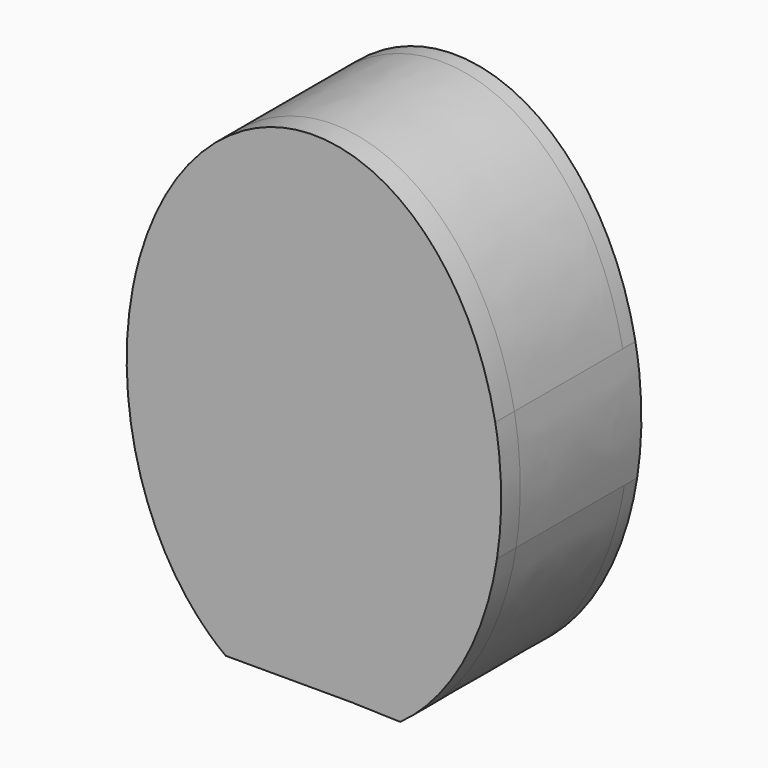
from build123d import *

# Parameters (mm, degrees)
F1_DEPTH = 2
F2_START = 2
F2_DEPTH = 17
F3_START = 19
F3_DEPTH = 3
F4_DEPTH = 22
F5_DEPTH = 1.9


# Not quite as in the source:
# - a feature names something its author has since deleted; it is built from what else it names


with BuildPart() as f1:
    # F0 (on Front) → F1 (new body)
    with BuildSketch(Plane.XZ):
        with BuildLine():
            ThreePointArc((22.615939659, -28.955879261), (25.4430057238, -23.4443332064), (29.5330586852, -18.7923541416))
            ThreePointArc((29.5330586852, -18.7923541416), (31.5285740741, -1.0914136246), (14.5694942222, 4.3578971054))
            ThreePointArc((14.5694942222, 4.3578971054), (10.2295706847, 0.7277849341), (6.5230501824, -3.5470666953))
            ThreePointArc((6.5230501824, -3.5470666953), (5.0741774638, -5.5394834496), (4.0740678087, -7.7908691019))
            ThreePointArc((4.0740678087, -7.7908691019), (2.9738142449, -8.0303676706), (2.3612100631, -7.0855747908))
            ThreePointArc((2.3612100631, -7.0855747908), (3.4264007601, -4.0400208243), (5.1113933333, -1.2885066571))
            ThreePointArc((5.1113933333, -1.2885066571), (8.6689265704, 3.4029198706), (13.299004455, 7.0399384822))
            ThreePointArc((13.299004455, 7.0399384822), (32.0541613054, 3.3946614198), (36.1678472728, -15.2633540456))
            ThreePointArc((36.1678472728, -15.2633540456), (31.3626226074, -22.0360379057), (26.9920754255, -29.0970398237))
            ThreePointArc((26.9920754255, -29.0970398237), (25.2131477889, -37.6146832372), (25.5804176451, -46.3083559771))
            Line((25.5804176451, -46.3083559771), (31.5964009875, -46.4919595582))
            add(Edge.make_bspline(
                [(31.5964009875, -46.4919595582), (41.4151881919, -39.4487656176), (43.7491179336, -24.5017576963)],
                knots=[0.4786752717, 0.4786752717, 0.4786752717, 1.3582145289, 1.3582145289, 1.3582145289], degree=2, weights=[1, 0.9048497635, 1]))
            Line((43.7491179336, -24.5017576963), (41.5137453779, -24.5017576963))
            Line((41.5137453779, -24.5017576963), (40.8978872001, -24.5017576963))
            Line((40.8978872001, -24.5017576963), (40.8978872001, -9.5017576963))
            Line((40.8978872001, -9.5017576963), (41.4988510311, -9.5017576963))
            Line((41.4988510311, -9.5017576963), (43.5284191526, -9.5017576963))
            add(Edge.make_bspline(
                [(43.5284191526, -9.5017576963), (38.9680565578, 14.8552314192), (20.7669530064, 14.8552314192), (2.5658494549, 14.8552314192), (-1.9945131398, -9.5017576963)],
                knots=[1.82404898, 1.82404898, 1.82404898, 3.1415926536, 3.1415926536, 4.4591363272, 4.4591363272, 4.4591363272], degree=2, weights=[1, 0.7907446431, 1, 0.7907446431, 1]))
            Line((-1.9945131398, -9.5017576963), (0, -9.5017576963))
            Line((0, -9.5017576963), (0.8074482903, -9.5017576963))
            Line((0.8074482903, -9.5017576963), (0.8074482903, -24.5017576963))
            Line((0.8074482903, -24.5017576963), (0, -24.5017576963))
            Line((0, -24.5017576963), (-2.2152119208, -24.5017576963))
            add(Edge.make_bspline(
                [(-2.2152119208, -24.5017576963), (0.0820950249, -39.2142250435), (9.6852980207, -46.3083559771)],
                knots=[4.9249707783, 4.9249707783, 4.9249707783, 5.7923862825, 5.7923862825, 5.7923862825], degree=2, weights=[1, 0.9074138517, 1]))
            Line((9.6852980207, -46.3083559771), (21.2042818786, -46.3083559771))
            ThreePointArc((21.2042818786, -46.3083559771), (21.3694737395, -37.5881357437), (22.615939659, -28.955879261))
        make_face()
        with BuildLine():
            ThreePointArc((14.5694942222, 4.3578971054), (31.5285740741, -1.0914136246), (29.5330586852, -18.7923541416))
            ThreePointArc((29.5330586852, -18.7923541416), (25.4430057238, -23.4443332064), (22.615939659, -28.955879261))
            ThreePointArc((22.615939659, -28.955879261), (21.3694737395, -37.5881357437), (21.2042818786, -46.3083559771))
            Line((21.2042818786, -46.3083559771), (25.5804176451, -46.3083559771))
            ThreePointArc((25.5804176451, -46.3083559771), (25.2131477889, -37.6146832372), (26.9920754255, -29.0970398237))
            ThreePointArc((26.9920754255, -29.0970398237), (31.3626226074, -22.0360379057), (36.1678472728, -15.2633540456))
            ThreePointArc((36.1678472728, -15.2633540456), (32.0541613054, 3.3946614198), (13.299004455, 7.0399384822))
            ThreePointArc((13.299004455, 7.0399384822), (8.6689265704, 3.4029198706), (5.1113933333, -1.2885066571))
            ThreePointArc((5.1113933333, -1.2885066571), (3.4264007601, -4.0400208243), (2.3612100631, -7.0855747908))
            ThreePointArc((2.3612100631, -7.0855747908), (2.9738142449, -8.0303676706), (4.0740678087, -7.7908691019))
            ThreePointArc((4.0740678087, -7.7908691019), (5.0741774638, -5.5394834496), (6.5230501824, -3.5470666953))
            ThreePointArc((6.5230501824, -3.5470666953), (10.2295706847, 0.7277849341), (14.5694942222, 4.3578971054))
        make_face()
    extrude(amount=F1_DEPTH)

    # F0 (on Front) → F2 (join)
    with BuildSketch(Plane.XZ.offset(F2_START)):
        with BuildLine():
            ThreePointArc((22.615939659, -28.955879261), (25.4430057238, -23.4443332064), (29.5330586852, -18.7923541416))
            ThreePointArc((29.5330586852, -18.7923541416), (31.5285740741, -1.0914136246), (14.5694942222, 4.3578971054))
            ThreePointArc((14.5694942222, 4.3578971054), (10.2295706847, 0.7277849341), (6.5230501824, -3.5470666953))
            ThreePointArc((6.5230501824, -3.5470666953), (5.0741774638, -5.5394834496), (4.0740678087, -7.7908691019))
            ThreePointArc((4.0740678087, -7.7908691019), (2.9738142449, -8.0303676706), (2.3612100631, -7.0855747908))
            ThreePointArc((2.3612100631, -7.0855747908), (3.4264007601, -4.0400208243), (5.1113933333, -1.2885066571))
            ThreePointArc((5.1113933333, -1.2885066571), (8.6689265704, 3.4029198706), (13.299004455, 7.0399384822))
            ThreePointArc((13.299004455, 7.0399384822), (32.0541613054, 3.3946614198), (36.1678472728, -15.2633540456))
            ThreePointArc((36.1678472728, -15.2633540456), (31.3626226074, -22.0360379057), (26.9920754255, -29.0970398237))
            ThreePointArc((26.9920754255, -29.0970398237), (25.2131477889, -37.6146832372), (25.5804176451, -46.3083559771))
            Line((25.5804176451, -46.3083559771), (31.5964009875, -46.4919595582))
            add(Edge.make_bspline(
                [(31.5964009875, -46.4919595582), (41.4151881919, -39.4487656176), (43.7491179336, -24.5017576963)],
                knots=[0.4786752717, 0.4786752717, 0.4786752717, 1.3582145289, 1.3582145289, 1.3582145289], degree=2, weights=[1, 0.9048497635, 1]))
            Line((43.7491179336, -24.5017576963), (41.5137453779, -24.5017576963))
            Line((41.5137453779, -24.5017576963), (40.8978872001, -24.5017576963))
            Line((40.8978872001, -24.5017576963), (40.8978872001, -9.5017576963))
            Line((40.8978872001, -9.5017576963), (41.4988510311, -9.5017576963))
            Line((41.4988510311, -9.5017576963), (43.5284191526, -9.5017576963))
            add(Edge.make_bspline(
                [(43.5284191526, -9.5017576963), (38.9680565578, 14.8552314192), (20.7669530064, 14.8552314192), (2.5658494549, 14.8552314192), (-1.9945131398, -9.5017576963)],
                knots=[1.82404898, 1.82404898, 1.82404898, 3.1415926536, 3.1415926536, 4.4591363272, 4.4591363272, 4.4591363272], degree=2, weights=[1, 0.7907446431, 1, 0.7907446431, 1]))
            Line((-1.9945131398, -9.5017576963), (0, -9.5017576963))
            Line((0, -9.5017576963), (0.8074482903, -9.5017576963))
            Line((0.8074482903, -9.5017576963), (0.8074482903, -24.5017576963))
            Line((0.8074482903, -24.5017576963), (0, -24.5017576963))
            Line((0, -24.5017576963), (-2.2152119208, -24.5017576963))
            add(Edge.make_bspline(
                [(-2.2152119208, -24.5017576963), (0.0820950249, -39.2142250435), (9.6852980207, -46.3083559771)],
                knots=[4.9249707783, 4.9249707783, 4.9249707783, 5.7923862825, 5.7923862825, 5.7923862825], degree=2, weights=[1, 0.9074138517, 1]))
            Line((9.6852980207, -46.3083559771), (21.2042818786, -46.3083559771))
            ThreePointArc((21.2042818786, -46.3083559771), (21.3694737395, -37.5881357437), (22.615939659, -28.955879261))
        make_face()
    extrude(amount=F2_DEPTH)


with BuildPart() as f3:
    # F0 (on Front) → F3 (new body)
    with BuildSketch(Plane.XZ.offset(F3_START)):
        with BuildLine():
            ThreePointArc((22.615939659, -28.955879261), (25.4430057238, -23.4443332064), (29.5330586852, -18.7923541416))
            ThreePointArc((29.5330586852, -18.7923541416), (31.5285740741, -1.0914136246), (14.5694942222, 4.3578971054))
            ThreePointArc((14.5694942222, 4.3578971054), (10.2295706847, 0.7277849341), (6.5230501824, -3.5470666953))
            ThreePointArc((6.5230501824, -3.5470666953), (5.0741774638, -5.5394834496), (4.0740678087, -7.7908691019))
            ThreePointArc((4.0740678087, -7.7908691019), (2.9738142449, -8.0303676706), (2.3612100631, -7.0855747908))
            ThreePointArc((2.3612100631, -7.0855747908), (3.4264007601, -4.0400208243), (5.1113933333, -1.2885066571))
            ThreePointArc((5.1113933333, -1.2885066571), (8.6689265704, 3.4029198706), (13.299004455, 7.0399384822))
            ThreePointArc((13.299004455, 7.0399384822), (32.0541613054, 3.3946614198), (36.1678472728, -15.2633540456))
            ThreePointArc((36.1678472728, -15.2633540456), (31.3626226074, -22.0360379057), (26.9920754255, -29.0970398237))
            ThreePointArc((26.9920754255, -29.0970398237), (25.2131477889, -37.6146832372), (25.5804176451, -46.3083559771))
            Line((25.5804176451, -46.3083559771), (31.5964009875, -46.4919595582))
            add(Edge.make_bspline(
                [(31.5964009875, -46.4919595582), (41.4151881919, -39.4487656176), (43.7491179336, -24.5017576963)],
                knots=[0.4786752717, 0.4786752717, 0.4786752717, 1.3582145289, 1.3582145289, 1.3582145289], degree=2, weights=[1, 0.9048497635, 1]))
            Line((43.7491179336, -24.5017576963), (41.5137453779, -24.5017576963))
            Line((41.5137453779, -24.5017576963), (40.8978872001, -24.5017576963))
            Line((40.8978872001, -24.5017576963), (40.8978872001, -9.5017576963))
            Line((40.8978872001, -9.5017576963), (41.4988510311, -9.5017576963))
            Line((41.4988510311, -9.5017576963), (43.5284191526, -9.5017576963))
            add(Edge.make_bspline(
                [(43.5284191526, -9.5017576963), (38.9680565578, 14.8552314192), (20.7669530064, 14.8552314192), (2.5658494549, 14.8552314192), (-1.9945131398, -9.5017576963)],
                knots=[1.82404898, 1.82404898, 1.82404898, 3.1415926536, 3.1415926536, 4.4591363272, 4.4591363272, 4.4591363272], degree=2, weights=[1, 0.7907446431, 1, 0.7907446431, 1]))
            Line((-1.9945131398, -9.5017576963), (0, -9.5017576963))
            Line((0, -9.5017576963), (0.8074482903, -9.5017576963))
            Line((0.8074482903, -9.5017576963), (0.8074482903, -24.5017576963))
            Line((0.8074482903, -24.5017576963), (0, -24.5017576963))
            Line((0, -24.5017576963), (-2.2152119208, -24.5017576963))
            add(Edge.make_bspline(
                [(-2.2152119208, -24.5017576963), (0.0820950249, -39.2142250435), (9.6852980207, -46.3083559771)],
                knots=[4.9249707783, 4.9249707783, 4.9249707783, 5.7923862825, 5.7923862825, 5.7923862825], degree=2, weights=[1, 0.9074138517, 1]))
            Line((9.6852980207, -46.3083559771), (21.2042818786, -46.3083559771))
            ThreePointArc((21.2042818786, -46.3083559771), (21.3694737395, -37.5881357437), (22.615939659, -28.955879261))
        make_face()
        with BuildLine():
            ThreePointArc((14.5694942222, 4.3578971054), (31.5285740741, -1.0914136246), (29.5330586852, -18.7923541416))
            ThreePointArc((29.5330586852, -18.7923541416), (25.4430057238, -23.4443332064), (22.615939659, -28.955879261))
            ThreePointArc((22.615939659, -28.955879261), (21.3694737395, -37.5881357437), (21.2042818786, -46.3083559771))
            Line((21.2042818786, -46.3083559771), (25.5804176451, -46.3083559771))
            ThreePointArc((25.5804176451, -46.3083559771), (25.2131477889, -37.6146832372), (26.9920754255, -29.0970398237))
            ThreePointArc((26.9920754255, -29.0970398237), (31.3626226074, -22.0360379057), (36.1678472728, -15.2633540456))
            ThreePointArc((36.1678472728, -15.2633540456), (32.0541613054, 3.3946614198), (13.299004455, 7.0399384822))
            ThreePointArc((13.299004455, 7.0399384822), (8.6689265704, 3.4029198706), (5.1113933333, -1.2885066571))
            ThreePointArc((5.1113933333, -1.2885066571), (3.4264007601, -4.0400208243), (2.3612100631, -7.0855747908))
            ThreePointArc((2.3612100631, -7.0855747908), (2.9738142449, -8.0303676706), (4.0740678087, -7.7908691019))
            ThreePointArc((4.0740678087, -7.7908691019), (5.0741774638, -5.5394834496), (6.5230501824, -3.5470666953))
            ThreePointArc((6.5230501824, -3.5470666953), (10.2295706847, 0.7277849341), (14.5694942222, 4.3578971054))
        make_face()
        with BuildLine():
            Line((40.8978872001, -24.5017576963), (41.5137453779, -24.5017576963))
            ThreePointArc((41.5137453779, -24.5017576963), (42.4025157736, -17.0008677912), (41.4988510311, -9.5017576963))
            Line((41.4988510311, -9.5017576963), (40.8978872001, -9.5017576963))
            Line((40.8978872001, -9.5017576963), (40.8978872001, -24.5017576963))
        make_face()
        with BuildLine():
            Line((41.5137453779, -24.5017576963), (43.7491179336, -24.5017576963))
            add(Edge.make_bspline(
                [(43.7491179336, -24.5017576963), (44.9258702836, -16.9655725309), (43.5284191526, -9.5017576963)],
                knots=[1.3582145289, 1.3582145289, 1.3582145289, 1.82404898, 1.82404898, 1.82404898], degree=2, weights=[1, 0.972997191, 1]))
            Line((43.5284191526, -9.5017576963), (41.4988510311, -9.5017576963))
            ThreePointArc((41.4988510311, -9.5017576963), (42.4025157736, -17.0008677912), (41.5137453779, -24.5017576963))
        make_face()
        with BuildLine():
            ThreePointArc((0, -9.5017576963), (-0.7605131059, -17.0017576963), (0, -24.5017576963))
            Line((0, -24.5017576963), (0.8074482903, -24.5017576963))
            Line((0.8074482903, -24.5017576963), (0.8074482903, -9.5017576963))
            Line((0.8074482903, -9.5017576963), (0, -9.5017576963))
        make_face()
        with BuildLine():
            add(Edge.make_bspline(
                [(-1.9945131398, -9.5017576963), (-3.3919642708, -16.9655725309), (-2.2152119208, -24.5017576963)],
                knots=[4.4591363272, 4.4591363272, 4.4591363272, 4.9249707783, 4.9249707783, 4.9249707783], degree=2, weights=[1, 0.972997191, 1]))
            Line((-2.2152119208, -24.5017576963), (0, -24.5017576963))
            ThreePointArc((0, -24.5017576963), (-0.7605131059, -17.0017576963), (0, -9.5017576963))
            Line((0, -9.5017576963), (-1.9945131398, -9.5017576963))
        make_face()
    extrude(amount=F3_DEPTH)

    # F0 (on Front) → F4 (join)
    with BuildSketch(Plane.XZ):
        with BuildLine():
            add(Edge.make_bspline(
                [(-1.9945131398, -9.5017576963), (-3.3919642708, -16.9655725309), (-2.2152119208, -24.5017576963)],
                knots=[4.4591363272, 4.4591363272, 4.4591363272, 4.9249707783, 4.9249707783, 4.9249707783], degree=2, weights=[1, 0.972997191, 1]))
            Line((-2.2152119208, -24.5017576963), (0, -24.5017576963))
            ThreePointArc((0, -24.5017576963), (-0.7605131059, -17.0017576963), (0, -9.5017576963))
            Line((0, -9.5017576963), (-1.9945131398, -9.5017576963))
        make_face()
        with BuildLine():
            Line((41.5137453779, -24.5017576963), (43.7491179336, -24.5017576963))
            add(Edge.make_bspline(
                [(43.7491179336, -24.5017576963), (44.9258702836, -16.9655725309), (43.5284191526, -9.5017576963)],
                knots=[1.3582145289, 1.3582145289, 1.3582145289, 1.82404898, 1.82404898, 1.82404898], degree=2, weights=[1, 0.972997191, 1]))
            Line((43.5284191526, -9.5017576963), (41.4988510311, -9.5017576963))
            ThreePointArc((41.4988510311, -9.5017576963), (42.4025157736, -17.0008677912), (41.5137453779, -24.5017576963))
        make_face()
    extrude(amount=F4_DEPTH)

    # F0 (on Front) → F5 (join)
    with BuildSketch(Plane.XZ):
        with BuildLine():
            ThreePointArc((0, -9.5017576963), (-0.7605131059, -17.0017576963), (0, -24.5017576963))
            Line((0, -24.5017576963), (0.8074482903, -24.5017576963))
            Line((0.8074482903, -24.5017576963), (0.8074482903, -9.5017576963))
            Line((0.8074482903, -9.5017576963), (0, -9.5017576963))
        make_face()
        with BuildLine():
            Line((40.8978872001, -24.5017576963), (41.5137453779, -24.5017576963))
            ThreePointArc((41.5137453779, -24.5017576963), (42.4025157736, -17.0008677912), (41.4988510311, -9.5017576963))
            Line((41.4988510311, -9.5017576963), (40.8978872001, -9.5017576963))
            Line((40.8978872001, -9.5017576963), (40.8978872001, -24.5017576963))
        make_face()
    extrude(amount=F5_DEPTH)


solid = Compound([f1.part, f3.part])
